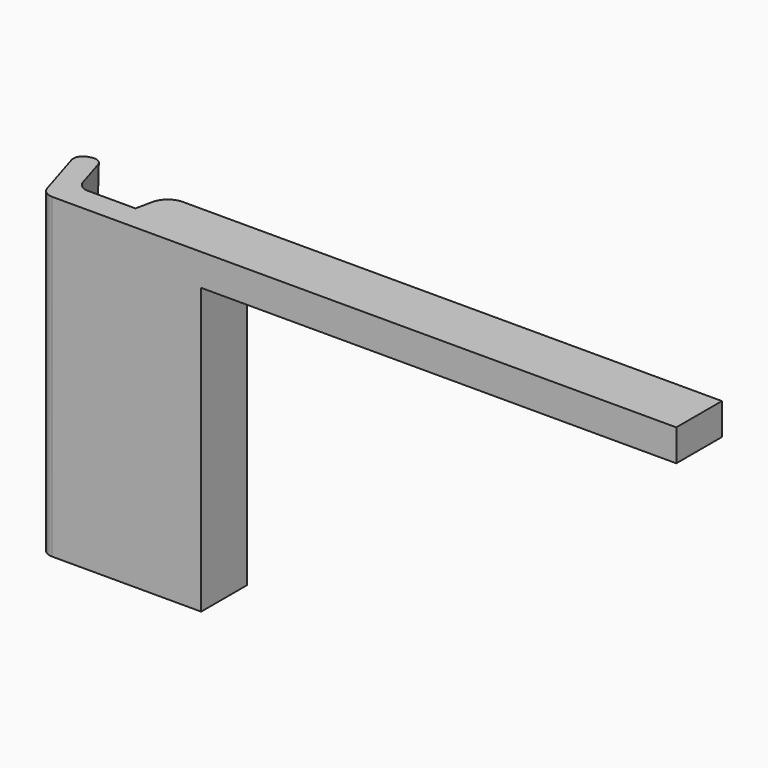
from build123d import *

# Parameters (mm, degrees)
F1_DEPTH    = 50
F2_SIZE2    = 2.99999
F2_SIZE     = 49.99999
F3_T1_DEPTH = 57.5899085645
F4_R        = 2
F5_R        = 3
F6_W        = 9
F6_H        = 5
F7_DEPTH    = 75
F8_R        = 2


# Not quite as in the source:
# - a fillet or chamfer that OpenCascade refuses, or shapes differently, is made with other operations: its cross-section is extruded or revolved along the edge and cut away or added
# - a fillet or chamfer is up to 0.001 mm smaller than in the source, because OpenCascade refuses the exact size


with BuildPart() as f1:
    # F0 (on Top) → F1 (new body)
    with BuildSketch(Plane.XY):
        Polygon((-4.3715766435, 7.6504380477), (-7.7186432894, 6.6271370812), (-4.4696014276, -4), (20.5303985724, -4), (20.5303985724, 5), (8.0088521886, 5), (6.9673969943, 0), (-2.0326030057, 0), align=None)
    extrude(amount=F1_DEPTH)

    # F2 (size 50 and 3 in the source; OpenCascade refuses exactly that, so slightly less here)
    f2_edges = [f1.edges().sort_by_distance(p)[0] for p in [
        (-6.04511, 7.138788, 0),
    ]]
    f2_side = f1.faces().sort_by_distance((-6.04511, 7.138788, 25))[0]
    chamfer(f2_edges, length=F2_SIZE, length2=F2_SIZE2, reference=f2_side)

    # F3: fillet of radius 1.5 on 2 edges, made by hand

    # F3_s2 → F3_t1 (cut)
    with BuildSketch(Plane(origin=(-0.948644568, 3.1028765694, 54.0777102773), x_dir=(0.956304756, 0.2923717047, 0), z_dir=(0.0175107565, -0.0572751036, -0.9982048567))):
        with BuildLine():
            ThreePointArc((-1.9437879213, -4.0842430614), (-2.3831277496, -5.1449032332), (-3.4437879213, -5.5842430614))
            Line((-3.4437879213, -5.5842430614), (-1.9437879213, -5.5842430614))
            Line((-1.9437879213, -5.5842430614), (-1.9437879213, -4.0842430614))
        make_face()
        with BuildLine():
            ThreePointArc((-3.9437879213, -5.5842430614), (-5.0044480931, -5.1449032332), (-5.4437879213, -4.0842430614))
            Line((-5.4437879213, -4.0842430614), (-5.4437879213, -5.5842430614))
            Line((-5.4437879213, -5.5842430614), (-3.9437879213, -5.5842430614))
        make_face()
    extrude(amount=F3_T1_DEPTH, mode=Mode.SUBTRACT)

    # F4
    f4_edges = [f1.edges().sort_by_distance(p)[0] for p in [
        (-2.032603, 0, 25),
    ]]
    fillet(f4_edges, radius=F4_R)

    # F5
    f5_edges = [f1.edges().sort_by_distance(p)[0] for p in [
        (8.008852, 5, 25),
    ]]
    fillet(f5_edges, radius=F5_R)

    # F6 (on face) → F7 (join)
    with BuildSketch(Plane.YZ.offset(20.5303985724)):
        with Locations((0.5, 47.5)):
            Rectangle(F6_W, F6_H)
    extrude(amount=F7_DEPTH)

    # F8
    f8_edges = [f1.edges().sort_by_distance(p)[0] for p in [
        (-4.469601, -4, 25),
    ]]
    fillet(f8_edges, radius=F8_R)


solid = f1.part
